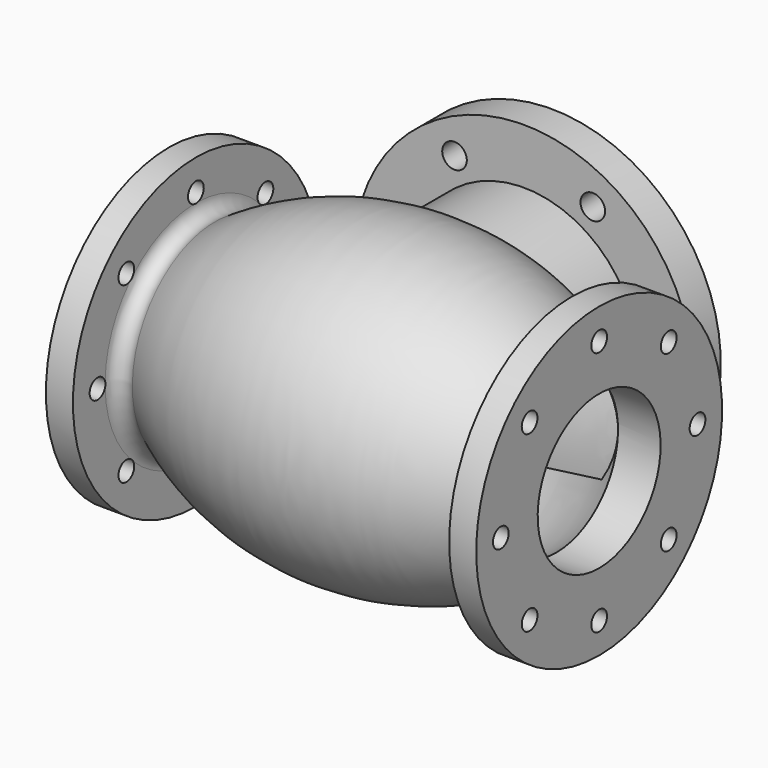
from build123d import *

# Parameters (mm, degrees)
F2_R           = 8
F3_DEPTH       = 25
F4_COUNT       = 8
F5_R           = 8
F6_DEPTH       = 25
F7_COUNT       = 8
F9_R           = 93
F9_R_2         = 85
F10_REACH      = 558.0447227014
F11_R          = 85
F12_DEPTH      = 125
F13_R          = 138
F13_R_2        = 93
F13_R_3        = 85
F14_DEPTH      = 28
F15_R          = 10
F16_DEPTH      = 28
F17_COUNT      = 6
F21_ANGLE_BACK = 20
F21_ANGLE      = 40


with BuildPart() as f1:
    # F0 (on Front) → F1 (revolve)
    with BuildSketch(Plane.XZ):
        with BuildLine():
            Line((175, -62.5), (175, 0))
            Line((175, 0), (140.3308590439, 0))
            ThreePointArc((140.3308590439, 0), (0, -46.5), (-140.3308590439, 0))
            Line((-140.3308590439, 0), (-175, 0))
            Line((-175, 0), (-175, -62.5))
            Line((-175, -62.5), (-153, -62.5))
            Line((-153, -62.5), (-153, -29.8391856722))
            ThreePointArc((-153, -29.8391856722), (-147.7545098575, -21.0417635489), (-137.5210727969, -21.4736996311))
            ThreePointArc((-137.5210727969, -21.4736996311), (0, -62.5), (137.5210727969, -21.4736996311))
            ThreePointArc((137.5210727969, -21.4736996311), (147.7545098575, -21.0417635489), (153, -29.8391856722))
            Line((153, -29.8391856722), (153, -62.5))
            Line((153, -62.5), (175, -62.5))
        make_face()
    revolve(axis=Axis((-27.7993068099, 0, 62.5), (1, 0, 0)))

    # F2 (on face) → F3 (cut)
    with BuildSketch(Plane.YZ.offset(175)):
        with Locations((0, 162.5)):
            Circle(F2_R)
    f3 = extrude(amount=-F3_DEPTH, mode=Mode.SUBTRACT)

    # F4: F3 ×8 about axis
    f4_axis = Axis((175, 0, 62.5), (1, 0, 0))
    for i in range(1, F4_COUNT):
        add(f3.rotate(f4_axis, i * 360 / F4_COUNT), mode=Mode.SUBTRACT)

    # F5 (on face) → F6 (cut)
    with BuildSketch(Plane(origin=(-175, 0, 0), x_dir=(0, -1, 0), z_dir=(-1, 0, 0))):
        with Locations((-100, 62.5)):
            Circle(F5_R)
    f6 = extrude(amount=-F6_DEPTH, mode=Mode.SUBTRACT)

    # F7: F6 ×8 about axis
    f7_axis = Axis((-175, 0, 62.5), (1, 0, 0))
    for i in range(1, F7_COUNT):
        add(f6.rotate(f7_axis, i * 360 / F7_COUNT), mode=Mode.SUBTRACT)

    f10_end = f1.faces().sort_by_distance((0, 0, 187.5))[0]
    # F9 (on offset) → F10 (join, up to a face of the model that its end follows)
    with BuildSketch(Plane.XZ.offset(-170)):
        with Locations((0, 65)):
            Circle(F9_R)
        with Locations((0, 65)):
            Circle(F9_R_2, mode=Mode.SUBTRACT)
    f10_long = extrude(amount=F10_REACH, mode=Mode.PRIVATE)
    add(split(f10_long, bisect_by=f10_end, keep=Keep.ALL, mode=Mode.PRIVATE).solids().sort_by_distance((-90.369562774, 170, 65))[0])

    # F11 (on face) → F12 (cut)
    with BuildSketch(Plane(origin=(0, 170, 0), x_dir=(-1, 0, 0), z_dir=(0, 1, 0))):
        with Locations((0, 65)):
            Circle(F11_R)
    extrude(amount=-F12_DEPTH, mode=Mode.SUBTRACT)

    # F13 (on face) → F14 (join)
    with BuildSketch(Plane(origin=(0, 170, 0), x_dir=(-1, 0, 0), z_dir=(0, 1, 0))):
        with Locations((0, 65)):
            Circle(F13_R)
        with Locations((0, 65)):
            Circle(F13_R_2, mode=Mode.SUBTRACT)
        with Locations((0, 65)):
            Circle(F13_R_2)
        with Locations((0, 65)):
            Circle(F13_R_3, mode=Mode.SUBTRACT)
    extrude(amount=-F14_DEPTH)

    # F15 (on face) → F16 (cut, through all)
    with BuildSketch(Plane(origin=(0, 170, 0), x_dir=(-1, 0, 0), z_dir=(0, 1, 0))):
        with Locations((-112.5, 65)):
            Circle(F15_R)
    f16 = extrude(amount=-F16_DEPTH, mode=Mode.SUBTRACT)

    # F17: F16 ×6 about axis
    f17_axis = Axis((0, 170, 65), (0, -1, 0))
    for i in range(1, F17_COUNT):
        add(f16.rotate(f17_axis, i * 360 / F17_COUNT), mode=Mode.SUBTRACT)

    # F20 (on line) → F21 (revolve)
    with BuildSketch(Plane(origin=(0, 0, 71.8713700771), x_dir=(1, 0, 0), z_dir=(0, 0, -1)), mode=Mode.PRIVATE) as f21_sk:
        Polygon((140.2069181204, -62.359880656), (88, -18.4656343404), (88, 50), (72, 50), (72, -15), (78, -15), (78, -25), (132.0858968386, -70.474043738), (140.5450195659, -62.6441477352), align=None)
        Polygon((-88, -25), (-78, -25), (-78, -15), (-72, -15), (-72, 38.6835938692), (-127.7431845665, 72.2227320075), (-141.0758048296, 62.8801584244), (-88, 30.2406232804), align=None)
    revolve(f21_sk.sketch.rotate(Axis((0, 170, 65), (0, 1, 0)), -F21_ANGLE_BACK), axis=Axis((0, 170, 65), (0, 1, 0)), revolution_arc=F21_ANGLE)


solid = f1.part
